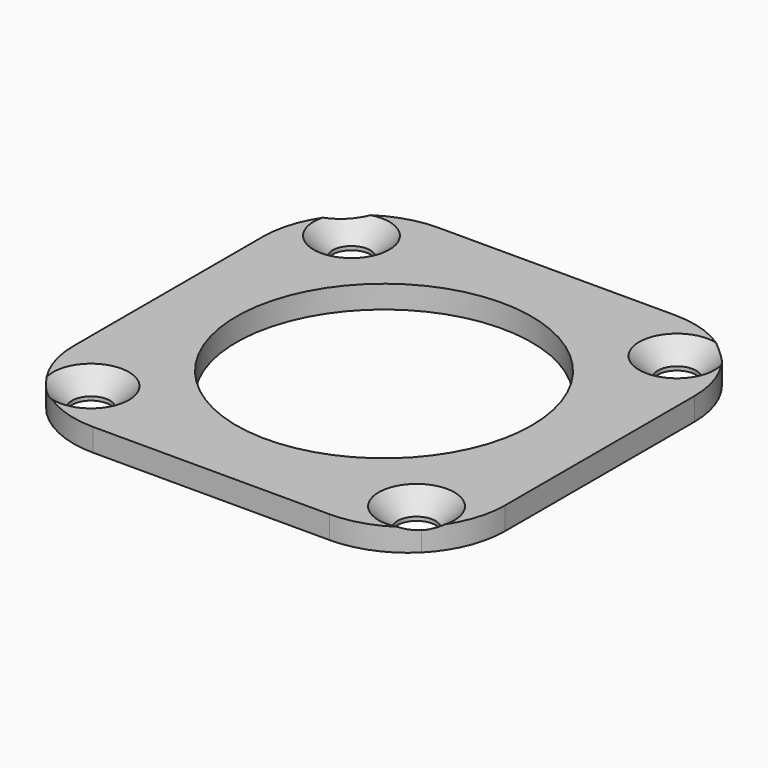
from build123d import *

# Parameters (mm, degrees)
F0_R        = 2.5
F0_R_2      = 23.5
F0_R_3      = 19.5
F1_DEPTH    = 3
F2_DEPTH    = 2.5
F3_T1_DEPTH = 32.6645215065


# Not quite as in the source:
# - a fillet or chamfer that OpenCascade refuses, or shapes differently, is made with other operations: its cross-section is extruded or revolved along the edge and cut away or added


with BuildPart() as f1:
    # F0 (on Top) → F1 (new body)
    with BuildSketch(Plane.XY):
        with BuildLine():
            Line((-20.3162496539, -28.5), (20.3162496539, -28.5))
            ThreePointArc((20.3162496539, -28.5), (24.7487373415, -24.7487373415), (28.5, -20.3162496539))
            Line((28.5, -20.3162496539), (28.5, 20.3162496539))
            ThreePointArc((28.5, 20.3162496539), (24.7487373415, 24.7487373415), (20.3162496539, 28.5))
            Line((20.3162496539, 28.5), (-20.3162496539, 28.5))
            ThreePointArc((-20.3162496539, 28.5), (-24.7487373415, 24.7487373415), (-28.5, 20.3162496539))
            Line((-28.5, 20.3162496539), (-28.5, -20.3162496539))
            ThreePointArc((-28.5, -20.3162496539), (-24.7487373415, -24.7487373415), (-20.3162496539, -28.5))
        make_face()
        with Locations((-21.5, -21.5)):
            Circle(F0_R, mode=Mode.SUBTRACT)
        with Locations((21.5, -21.5)):
            Circle(F0_R, mode=Mode.SUBTRACT)
        with Locations((-21.5, 21.5)):
            Circle(F0_R, mode=Mode.SUBTRACT)
        Circle(F0_R_2, mode=Mode.SUBTRACT)
        with Locations((21.5, 21.5)):
            Circle(F0_R, mode=Mode.SUBTRACT)
        Circle(F0_R_2)
        Circle(F0_R_3, mode=Mode.SUBTRACT)
    extrude(amount=F1_DEPTH)

    # F0 (on Top) → F2 (join)
    with BuildSketch(Plane.XY):
        Circle(F0_R_2)
        Circle(F0_R_3, mode=Mode.SUBTRACT)
    extrude(amount=F2_DEPTH)

    # F3: fillet of radius 13 on 8 edges, made by hand

    # F3_s2 → F3_t1 (cut)
    with BuildSketch(Plane.XY.offset(-14.8322607533)):
        with BuildLine():
            ThreePointArc((-28.5, 15.612494996), (-27.5014203705, 20.6090847421), (-24.6590909091, 24.8380602209))
            ThreePointArc((-24.6590909091, 24.8380602209), (-26.675530534, 22.6586864299), (-28.5, 20.3162496539))
            Line((-28.5, 20.3162496539), (-28.5, 15.612494996))
        make_face()
        with BuildLine():
            ThreePointArc((-24.8380602209, 24.6590909091), (-20.6090847421, 27.5014203705), (-15.612494996, 28.5))
            Line((-15.612494996, 28.5), (-20.3162496539, 28.5))
            ThreePointArc((-20.3162496539, 28.5), (-22.6586864299, 26.675530534), (-24.8380602209, 24.6590909091))
        make_face()
        with BuildLine():
            ThreePointArc((15.612494996, 28.5), (20.6090847421, 27.5014203705), (24.8380602209, 24.6590909091))
            ThreePointArc((24.8380602209, 24.6590909091), (22.6586864299, 26.675530534), (20.3162496539, 28.5))
            Line((20.3162496539, 28.5), (15.612494996, 28.5))
        make_face()
        with BuildLine():
            ThreePointArc((24.6590909091, 24.8380602209), (27.5014203705, 20.6090847421), (28.5, 15.612494996))
            Line((28.5, 15.612494996), (28.5, 20.3162496539))
            ThreePointArc((28.5, 20.3162496539), (26.675530534, 22.6586864299), (24.6590909091, 24.8380602209))
        make_face()
        with BuildLine():
            ThreePointArc((28.5, -15.612494996), (27.5014203705, -20.6090847421), (24.6590909091, -24.8380602209))
            ThreePointArc((24.6590909091, -24.8380602209), (26.675530534, -22.6586864299), (28.5, -20.3162496539))
            Line((28.5, -20.3162496539), (28.5, -15.612494996))
        make_face()
        with BuildLine():
            ThreePointArc((24.8380602209, -24.6590909091), (20.6090847421, -27.5014203705), (15.612494996, -28.5))
            Line((15.612494996, -28.5), (20.3162496539, -28.5))
            ThreePointArc((20.3162496539, -28.5), (22.6586864299, -26.675530534), (24.8380602209, -24.6590909091))
        make_face()
        with BuildLine():
            ThreePointArc((-24.8380602209, -24.6590909091), (-20.6090847421, -27.5014203705), (-15.612494996, -28.5))
            Line((-15.612494996, -28.5), (-20.3162496539, -28.5))
            ThreePointArc((-20.3162496539, -28.5), (-22.6586864299, -26.675530534), (-24.8380602209, -24.6590909091))
        make_face()
        with BuildLine():
            ThreePointArc((-24.6590909091, -24.8380602209), (-27.5014203705, -20.6090847421), (-28.5, -15.612494996))
            Line((-28.5, -15.612494996), (-28.5, -20.3162496539))
            ThreePointArc((-28.5, -20.3162496539), (-26.675530534, -22.6586864299), (-24.6590909091, -24.8380602209))
        make_face()
    extrude(amount=F3_T1_DEPTH, mode=Mode.SUBTRACT)

    # F4: chamfer of 2.5 on 4 edges, made by hand

    # F4_s1 → F4_t2 (revolve, cut)
    with BuildSketch(Plane.XZ.offset(-21.5)):
        Polygon((-16.5, 3), (-19, 0.5), (-19, 3), align=None)
    revolve(axis=Axis((-21.5, 21.5, 3), (0, 0, 1)), mode=Mode.SUBTRACT)

    # F4_s3 → F4_t4 (revolve, cut)
    with BuildSketch(Plane.XZ.offset(-21.5)):
        Polygon((26.5, 3), (24, 0.5), (24, 3), align=None)
    revolve(axis=Axis((21.5, 21.5, 3), (0, 0, 1)), mode=Mode.SUBTRACT)

    # F4_s5 → F4_t6 (revolve, cut)
    with BuildSketch(Plane.XZ.offset(21.5)):
        Polygon((26.5, 3), (24, 0.5), (24, 3), align=None)
    revolve(axis=Axis((21.5, -21.5, 3), (0, 0, 1)), mode=Mode.SUBTRACT)

    # F4_s7 → F4_t8 (revolve, cut)
    with BuildSketch(Plane.XZ.offset(21.5)):
        Polygon((-16.5, 3), (-19, 0.5), (-19, 3), align=None)
    revolve(axis=Axis((-21.5, -21.5, 3), (0, 0, 1)), mode=Mode.SUBTRACT)


solid = f1.part
